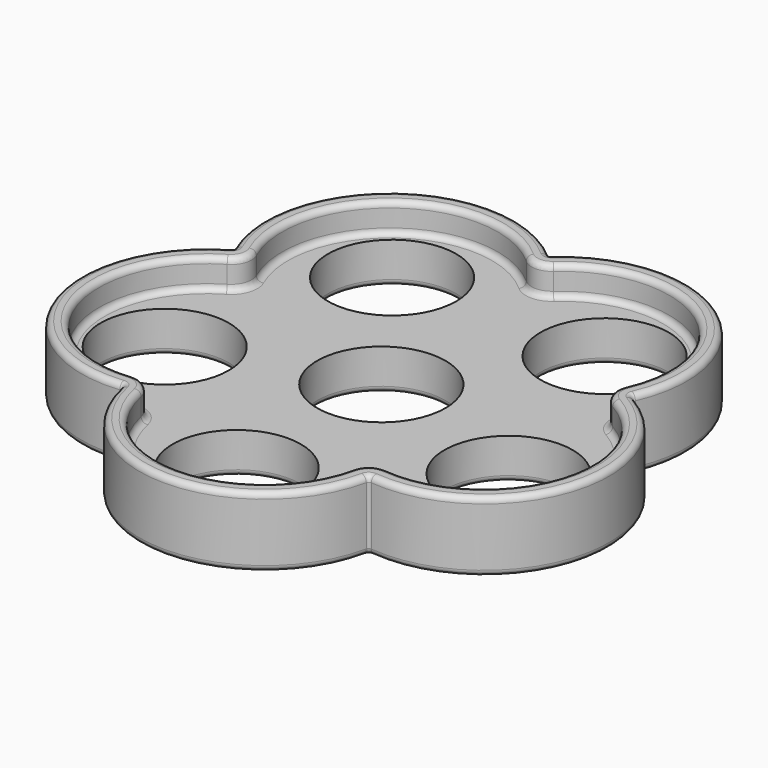
from build123d import *

# Parameters (mm, degrees)
F0_R     = 11
F1_DEPTH = 7
F2_R     = 2
F3_W     = 3
F3_H     = 12
F5_R     = 1


# Not quite as in the source:
# - two fillets or chamfers of one size are made in one step


with BuildPart() as f1:
    # F0 (on Top) → F1 (new body)
    with BuildSketch(Plane.XY):
        with BuildLine():
            ThreePointArc((32.1386573417, 10.4424827808), (26.4503363532, 36.4057647469), (0, 33.7925841325))
            ThreePointArc((0, 33.7925841325), (-26.4503363532, 36.4057647469), (-32.1386573417, 10.4424827808))
            ThreePointArc((-32.1386573417, 10.4424827808), (-42.7975432333, -13.9057647469), (-19.8627825899, -27.338774847))
            ThreePointArc((-19.8627825899, -27.338774847), (0, -45), (19.8627825899, -27.338774847))
            ThreePointArc((19.8627825899, -27.338774847), (42.7975432333, -13.9057647469), (32.1386573417, 10.4424827808))
        make_face()
        with Locations((0, -31)):
            Circle(F0_R, mode=Mode.SUBTRACT)
        with Locations((-29.4827520051, -9.5795268256)):
            Circle(F0_R, mode=Mode.SUBTRACT)
        with Locations((29.4827520051, -9.5795268256)):
            Circle(F0_R, mode=Mode.SUBTRACT)
        Circle(F0_R, mode=Mode.SUBTRACT)
        with Locations((-18.2213428211, 25.0795268256)):
            Circle(F0_R, mode=Mode.SUBTRACT)
        with Locations((18.2213428211, 25.0795268256)):
            Circle(F0_R, mode=Mode.SUBTRACT)
    extrude(amount=F1_DEPTH)

    # F2
    f2_edges = [f1.edges().sort_by_distance(p)[0] for p in [
        (19.862783, -27.338775, 3.5),
        (32.138657, 10.442483, 3.5),
        (0, 33.792584, 3.5),
        (-32.138657, 10.442483, 3.5),
        (-19.862783, -27.338775, 3.5),
    ]]
    fillet(f2_edges, radius=F2_R)

    # F4: sweep along a path in F4_path
    with BuildLine(Plane(origin=(19.5562572973, -29.1896062489, 7), x_dir=(0, -1, 0), z_dir=(0, 0, -1))) as f4_path:
        ThreePointArc((0, 0), (15.8103937511, 19.5562572973), (0, 39.1125145947))
        add(Plane(origin=(19.5562572973, -29.1896062489, 7), x_dir=(0, -1, 0), z_dir=(0, 0, -1)) * Edge.make_bspline(
            [(0, 39.1125145947), (-0.1096688398, 39.1360093386), (-0.2202265454, 39.167413391), (-0.3307214569, 39.2071742962), (-0.4400469579, 39.2555675645), (-0.5469942859, 39.3126073029), (-0.7548136485, 39.4440934015), (-0.8556175622, 39.5187164348), (-0.9515515376, 39.6015947804), (-1.0414196875, 39.6921471148), (-1.124187283, 39.789497972), (-1.2739594447, 39.9956416676), (-1.3409690183, 40.1044413979), (-1.3993186204, 40.2178932977), (-1.4484953823, 40.3347427474), (-1.488315982, 40.4536727518), (-1.549146978, 40.6919521499), (-1.5703464511, 40.8112913516), (-1.5825877465, 40.930220424), (-1.586257809, 41.0475941251), (-1.5819606279, 41.1624451373), (-1.5704159219, 41.2740066772)],
            knots=[0, 0, 0, 0, 0, 0, 0, 0.2487211213, 0.2487211213, 0.2487211213, 0.2487211213, 0.2487211213, 0.5, 0.5, 0.5, 0.5, 0.5, 0.7512788787, 0.7512788787, 0.7512788787, 0.7512788787, 0.7512788787, 1, 1, 1, 1, 1, 1, 1], degree=6))
        ThreePointArc((-1.5704159219, 41.2740066772), (-15.283841502, 62.3538005306), (-38.7686277958, 53.3604383796))
        add(Plane(origin=(19.5562572973, -29.1896062489, 7), x_dir=(0, -1, 0), z_dir=(0, 0, -1)) * Edge.make_bspline(
            [(-38.7686277958, 53.3604383796), (-38.8248621603, 53.2633973901), (-38.888893399, 53.1679551497), (-38.9608530724, 53.0751550394), (-39.0406612432, 52.9861346516), (-39.1279578, 52.902047947), (-39.3172282257, 52.7450314269), (-39.4193490702, 52.6722209934), (-39.5278162896, 52.6065931782), (-39.6417074628, 52.5491056988), (-39.7598702236, 52.5004721071), (-40.0022066718, 52.421732222), (-40.1263884613, 52.391623296), (-40.2523186486, 52.3711880918), (-40.3786455343, 52.3605266777), (-40.504059932, 52.3594064294), (-40.7494749178, 52.3751850976), (-40.8695242407, 52.391901042), (-40.9864152783, 52.4170099827), (-41.0991784132, 52.4497900143), (-41.2070803148, 52.489367791), (-41.3096141339, 52.5348218705)],
            knots=[0, 0, 0, 0, 0, 0, 0, 0.2487211213, 0.2487211213, 0.2487211213, 0.2487211213, 0.2487211213, 0.5, 0.5, 0.5, 0.5, 0.5, 0.7512788787, 0.7512788787, 0.7512788787, 0.7512788787, 0.7512788787, 1, 1, 1, 1, 1, 1, 1], degree=6))
        ThreePointArc((-41.3096141339, 52.5348218705), (-65.5953709957, 46.0065936505), (-64.2993733927, 20.8921328707))
        add(Plane(origin=(19.5562572973, -29.1896062489, 7), x_dir=(0, -1, 0), z_dir=(0, 0, -1)) * Edge.make_bspline(
            [(-64.2993733927, 20.8921328707), (-64.2244593015, 20.808663497), (-64.1534750778, 20.718272896), (-64.0874536902, 20.6211583685), (-64.0274523514, 20.5177474749), (-63.9744572626, 20.408739295), (-63.8836134561, 20.1802116502), (-63.8459236953, 20.0605892942), (-63.8170261481, 19.9371507283), (-63.7975466143, 19.8110691777), (-63.7878076212, 19.6836611078), (-63.7878076212, 19.4288534869), (-63.7975466143, 19.301445417), (-63.8170261481, 19.1753638664), (-63.8459236953, 19.0519253005), (-63.8836134561, 18.9323029445), (-63.9744572626, 18.7037752996), (-64.0274523514, 18.5947671198), (-64.0874536902, 18.4913562261), (-64.1534750778, 18.3942416987), (-64.2244593015, 18.3038510977), (-64.2993733927, 18.2203817239)],
            knots=[0, 0, 0, 0, 0, 0, 0, 0.2487211213, 0.2487211213, 0.2487211213, 0.2487211213, 0.2487211213, 0.5, 0.5, 0.5, 0.5, 0.5, 0.7512788787, 0.7512788787, 0.7512788787, 0.7512788787, 0.7512788787, 1, 1, 1, 1, 1, 1, 1], degree=6))
        ThreePointArc((-64.2993733927, 18.2203817239), (-65.5953709957, -6.8940790558), (-41.3096141339, -13.4223072759))
        add(Plane(origin=(19.5562572973, -29.1896062489, 7), x_dir=(0, -1, 0), z_dir=(0, 0, -1)) * Edge.make_bspline(
            [(-41.3096141339, -13.4223072759), (-41.2070803148, -13.3768531963), (-41.0991784132, -13.3372754196), (-40.9864152783, -13.3044953881), (-40.8695242407, -13.2793864474), (-40.7494749178, -13.2626705029), (-40.504059932, -13.2468918347), (-40.3786455343, -13.248012083), (-40.2523186486, -13.2586734971), (-40.1263884613, -13.2791087014), (-40.0022066718, -13.3092176273), (-39.7598702236, -13.3879575125), (-39.6417074628, -13.4365911042), (-39.5278162896, -13.4940785835), (-39.4193490702, -13.5597063987), (-39.3172282257, -13.6325168322), (-39.1279578, -13.7895333523), (-39.0406612432, -13.8736200569), (-38.9608530724, -13.9626404447), (-38.888893399, -14.055440555), (-38.8248621603, -14.1508827954), (-38.7686277958, -14.247923785)],
            knots=[0, 0, 0, 0, 0, 0, 0, 0.2487211213, 0.2487211213, 0.2487211213, 0.2487211213, 0.2487211213, 0.5, 0.5, 0.5, 0.5, 0.5, 0.7512788787, 0.7512788787, 0.7512788787, 0.7512788787, 0.7512788787, 1, 1, 1, 1, 1, 1, 1], degree=6))
        ThreePointArc((-38.7686277958, -14.247923785), (-15.283841502, -23.2412859359), (-1.5704159219, -2.1614920825))
        add(Plane(origin=(19.5562572973, -29.1896062489, 7), x_dir=(0, -1, 0), z_dir=(0, 0, -1)) * Edge.make_bspline(
            [(-1.5704159219, -2.1614920825), (-1.5819606279, -2.0499305426), (-1.586257809, -1.9350795304), (-1.5825877465, -1.8177058293), (-1.5703464511, -1.6987767569), (-1.549146978, -1.5794375553), (-1.488315982, -1.3411581572), (-1.4484953823, -1.2222281527), (-1.3993186204, -1.105378703), (-1.3409690183, -0.9919268033), (-1.2739594447, -0.883127073), (-1.124187283, -0.6769833773), (-1.0414196875, -0.5796325201), (-0.9515515376, -0.4890801857), (-0.8556175622, -0.4062018401), (-0.7548136485, -0.3315788068), (-0.5469942859, -0.2000927082), (-0.4400469579, -0.1430529698), (-0.3307214569, -0.0946597015), (-0.2202265454, -0.0548987964), (-0.1096688398, -0.0234947439), (0, 0)],
            knots=[0, 0, 0, 0, 0, 0, 0, 0.2487211213, 0.2487211213, 0.2487211213, 0.2487211213, 0.2487211213, 0.5, 0.5, 0.5, 0.5, 0.5, 0.7512788787, 0.7512788787, 0.7512788787, 0.7512788787, 0.7512788787, 1, 1, 1, 1, 1, 1, 1], degree=6))
    # F3 (on Right) → F4 (sweep)
    with BuildSketch(Plane.YZ):
        with Locations((-45, 6)):
            Rectangle(F3_W, F3_H)
    sweep(path=f4_path.line)

    # F5
    f5_edges = [f1.edges().sort_by_distance(p)[0] for p in [
        (0, -43.5, 12),
        (-19.454646, -26.777023, 12),
        (-41.370958, -13.442239, 12),
        (-31.478278, 10.227913, 12),
        (-25.568658, 35.192239, 12),
        (0, 33.098221, 12),
        (25.568658, 35.192239, 12),
        (31.478278, 10.227913, 12),
        (41.370958, -13.442239, 12),
        (19.454646, -26.777023, 12),
        (0, -46.5, 12),
        (21.217992, -29.204061, 12),
        (44.224128, -14.36929, 12),
        (34.331432, 11.154959, 12),
        (27.332014, 37.61929, 12),
        (0, 36.098204, 12),
        (-27.332014, 37.61929, 12),
        (-34.331432, 11.154959, 12),
        (-44.224128, -14.36929, 12),
        (-21.217992, -29.204061, 12),
        (21.022977, -29.503827, 6),
        (0, -46.5, 0),
        (-21.022977, -29.503827, 6),
        (21.217992, -29.204061, 0),
        (44.224128, -14.36929, 0),
        (34.331432, 11.154959, 0),
        (27.332014, 37.61929, 0),
        (0, 36.098204, 0),
        (-27.332014, 37.61929, 0),
        (-34.331432, 11.154959, 0),
        (-44.224128, -14.36929, 0),
        (-21.217992, -29.204061, 0),
        (18.482752, -9.579527, 0),
        (-11, 0, 0),
        (-29.221343, 25.079527, 0),
        (7.221343, 25.079527, 0),
        (-11, -31, 0),
        (-40.482752, -9.579527, 0),
        (-21.56335, -29.111223, 6),
        (-34.556264, 10.876855, 6),
        (-34.34986, 11.512102, 6),
        (-0.333969, 36.226093, 6),
        (0.333969, 36.226093, 6),
        (34.34986, 11.512102, 6),
        (34.556264, 10.876855, 6),
        (21.56335, -29.111223, 6),
        (-19.454646, -26.777023, 7),
        (-41.370958, -13.442239, 7),
        (-31.478278, 10.227913, 7),
        (-25.568658, 35.192239, 7),
        (0, 33.098221, 7),
        (25.568658, 35.192239, 7),
        (31.478278, 10.227913, 7),
        (41.370958, -13.442239, 7),
        (19.454646, -26.777023, 7),
        (0, -43.5, 7),
    ]]
    fillet(f5_edges, radius=F5_R)


solid = f1.part
